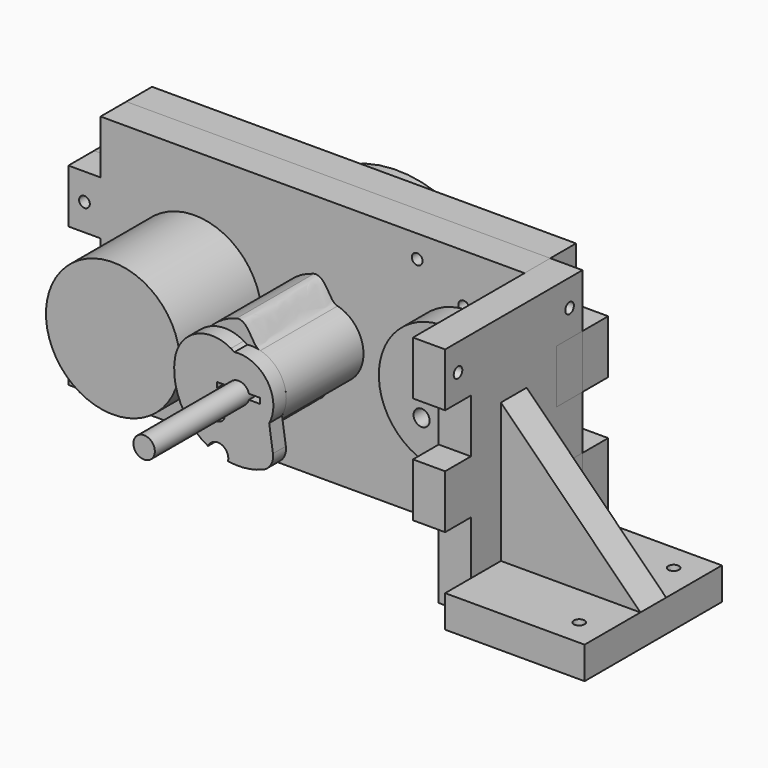
from build123d import *

# Parameters (mm, degrees)
F0_R      = 1.25
F0_R_2    = 6.5
F0_R_3    = 3.5
F0_R_4    = 1
F1_DEPTH  = 6
F6_R      = 1
F6_R_2    = 12.5
F6_R_3    = 2
F7_DEPTH  = 6
F8_D      = 2
F9_R      = 1.5
F10_DEPTH = 18
F11_W     = 6
F11_H     = 10
F11_R     = 1
F12_DEPTH = 6
F13_R     = 1
F13_W     = 10
F13_H     = 6
F14_DEPTH = 6
F16_DEPTH = 6
F17_R     = 1.5
F18_DEPTH = 3
F19_R     = 3
F20_R     = 7
F22_DEPTH = 42.001
F23_R     = 1.5
F24_DEPTH = 6


with BuildPart() as f1:
    # F0 (on Front) → F1 (new body)
    with BuildSketch(Plane.XZ):
        Polygon((36.5209371471, 13), (36.5209371471, 23), (-42.5209371471, 23), (-42.5209371471, 13), (-48.5209371471, 13), (-48.5209371471, 3), (-42.5209371471, 3), (-42.5209371471, -7), (-48.5209371471, -7), (-48.5209371471, -23), (42.5209371471, -23), (42.5209371471, -7), (36.5209371471, -7), (36.5209371471, 3), (42.5209371471, 3), (42.5209371471, 13), align=None)
        with Locations((-25, -8.75)):
            Circle(F0_R, mode=Mode.SUBTRACT)
        with Locations((-25, 0)):
            Circle(F0_R_2, mode=Mode.SUBTRACT)
        with Locations((-25, 8.75)):
            Circle(F0_R, mode=Mode.SUBTRACT)
        Circle(F0_R_3, mode=Mode.SUBTRACT)
        with Locations((16.5086770278, 18.7806704564)):
            Circle(F0_R_4, mode=Mode.SUBTRACT)
        with Locations((25.1879223108, 13.8137094824)):
            Circle(F0_R_4, mode=Mode.SUBTRACT)
    extrude(amount=F1_DEPTH)

    # F8 (through all)
    with Locations(Plane.XZ.offset(6)):
        with Locations((39.5209371471, 8), (39.5209371471, -15), (-45.5209371471, -15), (-45.5209371471, 8)):
            Hole(F8_D / 2)


with BuildPart() as f3:
    # F2 (on Top) → F3 (revolve)
    with BuildSketch(Plane.XY):
        Polygon((10, 9), (0, 9), (0, -55), (2, -55), (2, 0), (21.5, 0), (21.5, 4), (10, 4), align=None)
    revolve(axis=Axis((0, -23, 0), (0, -1, 0)))


with BuildPart() as f5:
    # F4 (on Top) → F5 (revolve)
    with BuildSketch(Plane.XY):
        Polygon((-25, -31), (-12.5, -31), (-12.5, -6), (-23, -6), (-23, 0), (-20.5, 0), (-20.5, 6), (-25, 6), align=None)
    revolve(axis=Axis((-25, -12.5, 0), (0, -1, 0)))


with BuildPart() as f7:
    # F6 (on face) → F7 (new body)
    with BuildSketch(Plane.XZ.offset(6)):
        Polygon((36.5209371471, 13), (36.5209371471, 23), (-42.5209371471, 23), (-42.5209371471, 13), (-48.5209371471, 13), (-48.5209371471, 3), (-42.5209371471, 3), (-42.5209371471, -7), (-48.5209371471, -7), (-48.5209371471, -23), (42.5209371471, -23), (42.5209371471, -7), (36.5209371471, -7), (36.5209371471, 3), (42.5209371471, 3), (42.5209371471, 13), align=None)
        with Locations((-45.5209371471, -15)):
            Circle(F6_R, mode=Mode.SUBTRACT)
        with Locations((39.5209371471, -15)):
            Circle(F6_R, mode=Mode.SUBTRACT)
        with Locations((-45.5209371471, 8)):
            Circle(F6_R, mode=Mode.SUBTRACT)
        with Locations((-25, 0)):
            Circle(F6_R_2, mode=Mode.SUBTRACT)
        Circle(F6_R_3, mode=Mode.SUBTRACT)
        with Locations((39.5209371471, 8)):
            Circle(F6_R, mode=Mode.SUBTRACT)
        with Locations((16.5086770278, 18.7806704564)):
            Circle(F6_R, mode=Mode.SUBTRACT)
        with Locations((25.1879223108, 13.8137094824)):
            Circle(F6_R, mode=Mode.SUBTRACT)
    extrude(amount=F7_DEPTH)


with BuildPart() as f10:
    # F9 (on face) → F10 (new body)
    with BuildSketch(Plane.XZ.offset(12)):
        with BuildLine():
            add(Edge.make_bspline(
                [(-2.7175999736, -10.142221176), (-0.3785296212, -10.493174702), (0.0260690487, -6.4999477232), (1.6823237932, -6.2785178709)],
                knots=[0, 0, 0, 0, 5.8555556853, 5.8555556853, 5.8555556853, 5.8555556853], degree=3))
            ThreePointArc((1.6823237932, -6.2785178709), (6.5, 0), (1.6823237932, 6.2785178709))
            add(Edge.make_bspline(
                [(-2.7175999736, 10.142221176), (-0.3785296212, 10.493174702), (0.0260690487, 6.4999477232), (1.6823237932, 6.2785178709)],
                knots=[0, 0, 0, 0, 5.8555556853, 5.8555556853, 5.8555556853, 5.8555556853], degree=3))
            ThreePointArc((-2.7175999736, 10.142221176), (-10.5, 0), (-2.7175999736, -10.142221176))
        make_face()
        with Locations((-6, 0)):
            Circle(F9_R, mode=Mode.SUBTRACT)
        with BuildLine():
            ThreePointArc((1.9364916731, -0.5), (0, -2), (-1.9364916731, -0.5))
            Line((-1.9364916731, -0.5), (-4, -0.5))
            Line((-4, -0.5), (-4, 0.5))
            Line((-4, 0.5), (-1.9364916731, 0.5))
            ThreePointArc((-1.9364916731, 0.5), (0, 2), (1.9364916731, 0.5))
            Line((1.9364916731, 0.5), (4, 0.5))
            Line((4, 0.5), (4, -0.5))
            Line((4, -0.5), (1.9364916731, -0.5))
        make_face(mode=Mode.SUBTRACT)
    extrude(amount=F10_DEPTH)


with BuildPart() as f12:
    # F11 (on face) → F12 (new body)
    with BuildSketch(Plane.YZ.offset(36.5209371471)):
        Polygon((-6, 13), (-6, 23), (-22, 23), (-38, 23), (-38, 13), (-32, 13), (-32, 3), (-38, 3), (-38, -7), (-32, -7), (-32, -23), (-25, -23), (-25, -17), (-22, -17), (-19, -17), (-19, -23), (-12, -23), (-12, -7), (-6, -7), (-6, 3), (-12, 3), (-12, 13), align=None)
        with Locations((-22, -2)):
            Rectangle(F11_W, F11_H, mode=Mode.SUBTRACT)
        with Locations((-35, 18)):
            Circle(F11_R, mode=Mode.SUBTRACT)
        with Locations((-9, 18)):
            Circle(F11_R, mode=Mode.SUBTRACT)
    extrude(amount=F12_DEPTH)


with BuildPart() as f14:
    # F13 (on face) → F14 (new body)
    with BuildSketch(Plane(origin=(0, 0, -17), x_dir=(1, 0, 0), z_dir=(0, 0, -1))):
        Polygon((42.5209371471, 38), (42.5209371471, 25), (36.5209371471, 25), (36.5209371471, 19), (42.5209371471, 19), (42.5209371471, 6), (68.5209371471, 6), (68.5209371471, 38), align=None)
        with Locations((63.5209371471, 11)):
            Circle(F13_R, mode=Mode.SUBTRACT)
        with Locations((57.5209371471, 22)):
            Rectangle(F13_W, F13_H, mode=Mode.SUBTRACT)
        with Locations((63.5209371471, 33)):
            Circle(F13_R, mode=Mode.SUBTRACT)
    extrude(amount=F14_DEPTH)


with BuildPart() as f16:
    # F15 (on face) → F16 (new body)
    with BuildSketch(Plane.XZ.offset(19)):
        Polygon((62.5209371471, -17), (68.5209371471, -17), (42.5209371471, 9), (42.5209371471, 3), (36.5209371471, 3), (36.5209371471, -7), (42.5209371471, -7), (42.5209371471, -17), (52.5209371471, -17), (52.5209371471, -23), (62.5209371471, -23), align=None)
    extrude(amount=F16_DEPTH)


with BuildPart() as f18:
    # F17 (on face) → F18 (new body)
    with BuildSketch(Plane.XZ.offset(30)):
        with BuildLine():
            Line((-0.7459832887, 6.4570511019), (-6.7236078935, 9.9394716607))
            ThreePointArc((-6.7236078935, 9.9394716607), (-9.9394716607, -6.7236078935), (6.7236078935, -9.9394716607))
            Line((6.7236078935, -9.9394716607), (5.7157191191, -3.0952471552))
            ThreePointArc((5.7157191191, -3.0952471552), (5.3838804829, 3.6419542756), (-0.7459832887, 6.4570511019))
        make_face()
        with Locations((-4.0242874639, -4.4502932946)):
            Circle(F17_R, mode=Mode.SUBTRACT)
        with BuildLine():
            Line((-4, -0.5), (-4, 0.5))
            Line((-4, 0.5), (-1.9364916731, 0.5))
            ThreePointArc((-1.9364916731, 0.5), (0, 2), (1.9364916731, 0.5))
            Line((1.9364916731, 0.5), (4, 0.5))
            Line((4, 0.5), (4, -0.5))
            Line((4, -0.5), (1.9364916731, -0.5))
            ThreePointArc((1.9364916731, -0.5), (0, -2), (-1.9364916731, -0.5))
            Line((-1.9364916731, -0.5), (-4, -0.5))
        make_face(mode=Mode.SUBTRACT)
    extrude(amount=F18_DEPTH)

    # F19
    f19_edges = [f18.edges().sort_by_distance(p)[0] for p in [
        (6.723608, -31.5, -9.939472),
    ]]
    fillet(f19_edges, radius=F19_R)

    # F20
    f20_edges = [f18.edges().sort_by_distance(p)[0] for p in [
        (-6.723608, -31.5, 9.939472),
    ]]
    fillet(f20_edges, radius=F20_R)

    # F21 (on face) → F22 (cut, through all)
    with BuildSketch(Plane.XZ.offset(33)):
        with BuildLine():
            ThreePointArc((-5.69120253, -10.5645735249), (-3.8802280805, -11.3553436779), (-1.9640308484, -11.838183257))
            ThreePointArc((-1.9640308484, -11.838183257), (-3.2412535928, -9.4854085197), (-5.69120253, -10.5645735249))
        make_face()
    extrude(amount=-F22_DEPTH, mode=Mode.SUBTRACT)


with BuildPart() as f24:
    # F23 (on face) → F24 (new body)
    with BuildSketch(Plane.XZ.offset(12)):
        with BuildLine():
            ThreePointArc((29.8785366044, 10.7458675016), (28.8182674664, 11.7398437475), (28.7108556093, 13.1891960564))
            ThreePointArc((28.7108556093, 13.1891960564), (14.4871210247, -1.3300751794), (33.7441280678, -7.8332699709))
            ThreePointArc((33.7441280678, -7.8332699709), (33.1835017989, -6.492427844), (33.6786464482, -5.1260489805))
            ThreePointArc((33.6786464482, -5.1260489805), (35.8824375063, 3.7924664409), (29.8785366044, 10.7458675016))
        make_face()
        with Locations((22.1330061871, -2.9862548629)):
            Circle(F23_R, mode=Mode.SUBTRACT)
        with BuildLine():
            Line((22.157293651, 0.9640384317), (22.157293651, 1.9640384317))
            Line((22.157293651, 1.9640384317), (24.2208019779, 1.9640384317))
            ThreePointArc((24.2208019779, 1.9640384317), (26.157293651, 3.4640384317), (28.0937853241, 1.9640384317))
            Line((28.0937853241, 1.9640384317), (30.157293651, 1.9640384317))
            Line((30.157293651, 1.9640384317), (30.157293651, 0.9640384317))
            Line((30.157293651, 0.9640384317), (28.0937853241, 0.9640384317))
            ThreePointArc((28.0937853241, 0.9640384317), (26.157293651, -0.5359615683), (24.2208019779, 0.9640384317))
            Line((24.2208019779, 0.9640384317), (22.157293651, 0.9640384317))
        make_face(mode=Mode.SUBTRACT)
    extrude(amount=F24_DEPTH)


solid = Compound([f1.part, f3.part, f5.part, f7.part, f10.part, f12.part, f14.part, f16.part, f18.part, f24.part])
